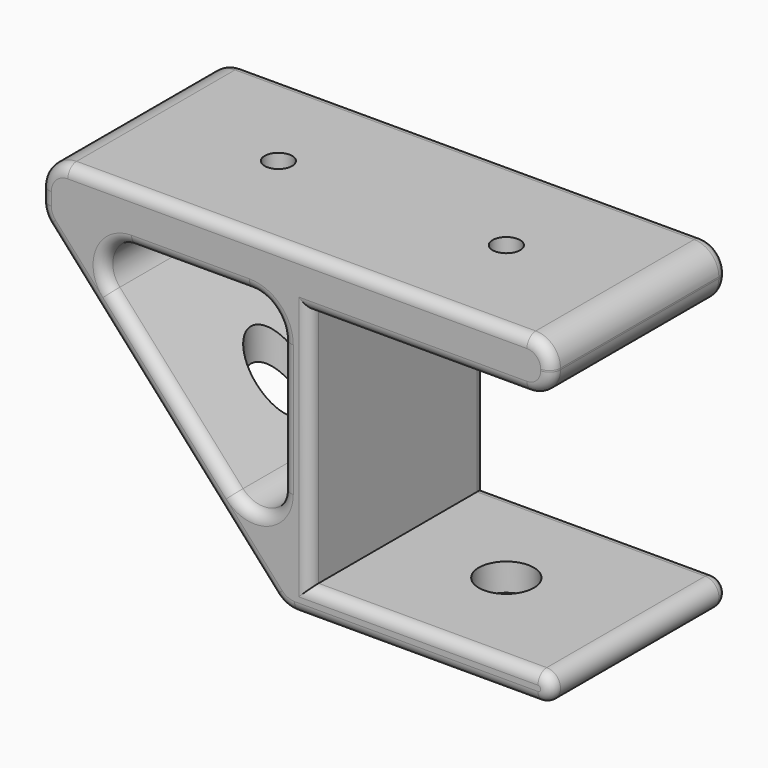
from build123d import *

# Parameters (mm, degrees)
F1_DEPTH             = 20
F2_R                 = 5
F3_R                 = 1.99999
F6_D                 = 5
F6_DEPTH             = 10
F6_CSINK_D           = 10
F6_CSINK_ANGLE       = 90
F6_TIP               = 1.5021515476
F6_ON_F5_D           = 5
F6_ON_F5_DEPTH       = 10
F6_ON_F5_CSINK_D     = 10
F6_ON_F5_CSINK_ANGLE = 90
F6_ON_F5_TIP         = 1.5021515476
F7_D                 = 10
F7_DEPTH             = 49.0010001
F7_ON_F5_D           = 10
F7_ON_F5_DEPTH       = 49.0010001


# Not quite as in the source:
# - a fillet or chamfer is up to 0.001 mm smaller than in the source, because OpenCascade refuses the exact size


with BuildPart() as f1:
    # F0 (on Front) → F1 (new body, symmetric)
    with BuildSketch(Plane.XZ):
        with BuildLine():
            Line((44.5, 0), (-44, 0))
            Line((-44, 0), (-44, -9.25))
            Line((-44, -9.25), (0, -58.25))
            Line((0, -58.25), (46.5, -58.25))
            ThreePointArc((46.5, -58.25), (48.267766953, -57.517766953), (49, -55.75))
            ThreePointArc((49, -55.75), (48.267766953, -53.982233047), (46.5, -53.25))
            Line((46.5, -53.25), (5, -53.25))
            Line((5, -53.25), (5, -9.25))
            Line((5, -9.25), (44.5, -9.25))
            ThreePointArc((44.5, -9.25), (47.6819805153, -7.9319805153), (49, -4.75))
            Line((49, -4.75), (49, -4.5))
            ThreePointArc((49, -4.5), (47.6819805153, -1.3180194847), (44.5, 0))
        make_face()
        with BuildLine():
            Line((0, -52.2630996996), (-38.6240078935, -9.25))
            Line((-38.6240078935, -9.25), (-6, -9.25))
            ThreePointArc((-6, -9.25), (-1.7573593129, -11.0073593129), (0, -15.25))
            Line((0, -15.25), (0, -52.2630996996))
        make_face(mode=Mode.SUBTRACT)
    extrude(amount=F1_DEPTH, both=True)

    # F2
    f2_edges = [f1.edges().sort_by_distance(p)[0] for p in [
        (-44, 0, 0),
        (-44, 0, -9.25),
        (-38.624008, 0, -9.25),
        (0, 0, -52.2631),
        (0, 0, -58.25),
    ]]
    fillet(f2_edges, radius=F2_R)

    # F3 (radius 2 in the source; OpenCascade refuses exactly that, so slightly less here)
    f3_edges = [f1.edges().sort_by_distance(p)[0] for p in [
        (24.75, -20, -9.25),
        (25.75, -20, -53.25),
        (24.75, 20, -9.25),
        (-16.707111, -20, -9.25),
        (5, -20, -31.25),
        (5, 20, -31.25),
        (-16.707111, 20, -9.25),
    ]]
    fillet(f3_edges, radius=F3_R)

    # F6
    with Locations(Plane(origin=(0, 0, -9.25), x_dir=(1, 0, 0), z_dir=(0, 0, -1))):
        with Locations((24.75, 0)):
            CounterSinkHole(F6_D / 2, F6_CSINK_D / 2, depth=F6_DEPTH, counter_sink_angle=F6_CSINK_ANGLE)
            with Locations((0, 0, -(F6_DEPTH + F6_TIP / 2))):  # 118° drill point
                Cone(0, F6_D / 2, F6_TIP, mode=Mode.SUBTRACT)

    # F6 on F5
    with Locations(Plane(origin=(0, 0, -9.25), x_dir=(1, 0, 0), z_dir=(0, 0, -1))):
        with Locations((-16.7071109211, 0)):
            CounterSinkHole(F6_ON_F5_D / 2, F6_ON_F5_CSINK_D / 2, depth=F6_ON_F5_DEPTH, counter_sink_angle=F6_ON_F5_CSINK_ANGLE)
            with Locations((0, 0, -(F6_ON_F5_DEPTH + F6_ON_F5_TIP / 2))):  # 118° drill point
                Cone(0, F6_ON_F5_D / 2, F6_ON_F5_TIP, mode=Mode.SUBTRACT)

    # F7 (through all, one way)
    with BuildSketch(Plane.XY.offset(-9.25)):
        with Locations((24.75, 0)):
            Circle(F7_D / 2)
    extrude(amount=-F7_DEPTH, mode=Mode.SUBTRACT)

    # F7 on F5 (through all, one way)
    with BuildSketch(Plane.XY.offset(-9.25)):
        with Locations((-16.7071109211, 0)):
            Circle(F7_ON_F5_D / 2)
    extrude(amount=-F7_ON_F5_DEPTH, mode=Mode.SUBTRACT)


solid = f1.part
